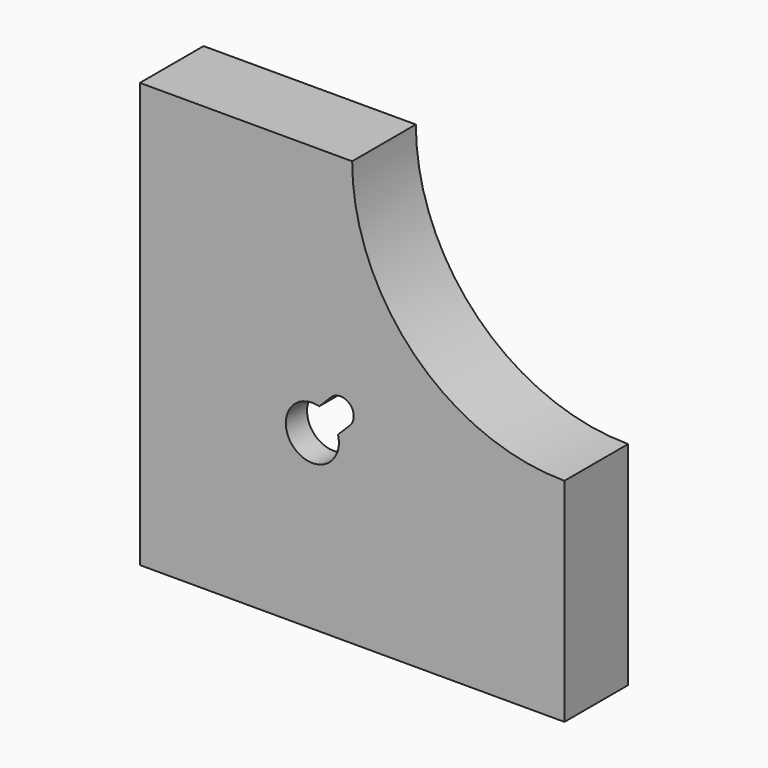
from build123d import *

# Parameters (mm, degrees)
F9_DEPTH      = 3.175
F9_DEPTH_BACK = 6.35
F7_R          = 3.175
F10_DEPTH     = 3.176
F3_R          = 13.0054161967
F4_R          = 1.5875
F11_DEPTH     = 6.351


# Not quite as in the source:
# - a variable given as a bare number and used for a length is read in inches; the dataset says mm whatever the document's units were


with BuildPart() as f9:
    # F1 (on Front) → F9 (new body, two sides)
    with BuildSketch(Plane.XZ) as f9_sk:
        with BuildLine():
            Line((0, 50.8), (0, 0))
            Line((0, 0), (50.8, 0))
            Line((50.8, 0), (50.8, 25.4))
            ThreePointArc((50.8, 25.4), (32.8394877579, 32.8394877579), (25.4, 50.8))
            Line((25.4, 50.8), (0, 50.8))
        make_face()
    extrude(amount=F9_DEPTH)
    extrude(f9_sk.sketch, amount=-F9_DEPTH_BACK)

    # F8 (on Front) + F7 (on Front) → F10 (cut, through all)
    with BuildSketch(Plane.XZ):
        with BuildLine():
            Line((22.8825640303, 25.1276280605), (21.4592504682, 23.7043144985))
            Line((21.4592504682, 23.7043144985), (23.7043144985, 21.4592504682))
            Line((23.7043144985, 21.4592504682), (25.1276280605, 22.8825640303))
            ThreePointArc((25.1276280605, 22.8825640303), (25.1276280605, 25.1276280605), (22.8825640303, 25.1276280605))
        make_face()
    with BuildSketch(Plane.XZ):
        with Locations((20.6375, 20.6375)):
            Circle(F7_R)
    extrude(amount=F10_DEPTH, mode=Mode.SUBTRACT)

    # F3 (on Front) + F4 (on Front) + F6 (on face) → F11 (cut, through all)
    with BuildSketch(Plane.XZ):
        with Locations((20.6375, 20.6375)):
            Circle(F3_R)
    with BuildSketch(Plane.XZ):
        with Locations((37.4589580984, 20.6375)):
            Circle(F4_R)
        with Locations((20.6375, 37.4589580984)):
            Circle(F4_R)
        with Locations((5.159375, 5.159375)):
            Circle(F4_R)
    with BuildSketch(Plane.XZ):
        Polygon((17.0707799442, 8.1307274949), (13.0054161967, 0), (28.2695838033, 0), (24.7028637475, 8.1307274949), align=None)
        Polygon((8.1307274949, 24.7028637475), (0, 28.2695838033), (0, 13.0054161967), (8.1307274949, 17.0707799442), align=None)
    extrude(amount=-F11_DEPTH, mode=Mode.SUBTRACT)


solid = f9.part
